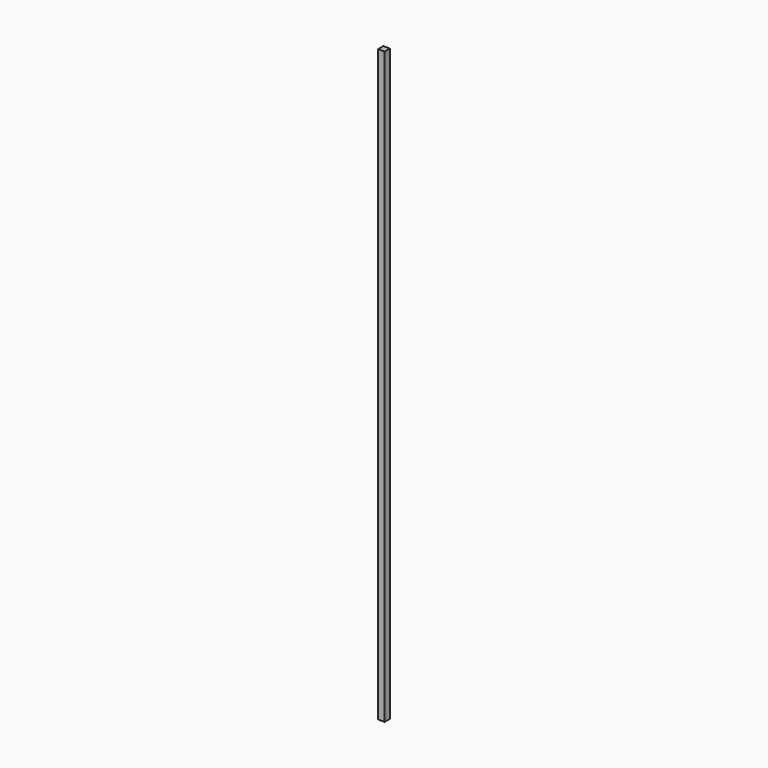
from build123d import *

# Parameters (mm, degrees)
F0_W     = 40
F0_H     = 40
F1_DEPTH = 1800
F2_DEPTH = 1800.8986695


# Not quite as in the source:
# - an extrude ends at something that could not be found from the text; its depth is read off the source's solid


with BuildPart() as f1:
    # F0 (on Top) → F1 (new body)
    with BuildSketch(Plane.XY):
        Rectangle(F0_W, F0_H)
    extrude(amount=F1_DEPTH)

    # F2 (add, through all): a face of the model
    f2_faces = [f1.faces().sort_by_distance(p)[0] for p in [
        (0, 0, 0),
    ]]
    extrude(f2_faces, amount=F2_DEPTH)


solid = f1.part
